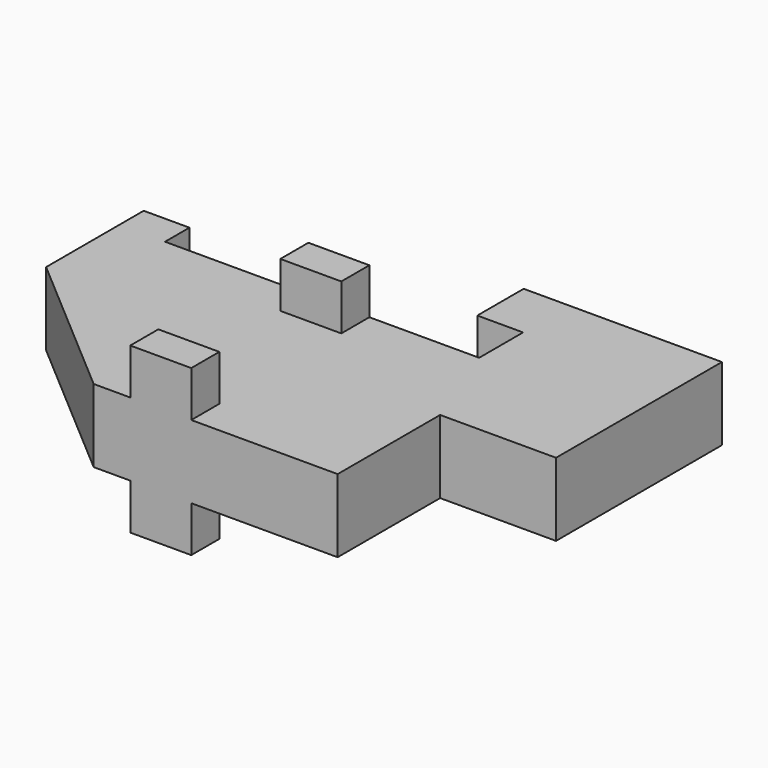
from build123d import *

# Parameters (mm, degrees)
F1_DEPTH = 1.2
F2_W     = 2
F2_H     = 1.15
F3_DEPTH = 1.5


# Not quite as in the source:
# - a pattern or mirror of a feature is missing from the dataset's text; its kind, count and spacing are read off the source's solid


with BuildPart() as f1:
    # F0 (on Top) → F1 (new body, symmetric)
    with BuildSketch(Plane.XY):
        Polygon((0, 4.2), (0, 11), (-6.5, 11), (-6.5, 9.1), (-5, 9.1), (-5, 7.3), (-15.3, 7.3), (-15.3, 8.3), (-16.8, 8.3), (-16.8, 4.3), (-11.8, 0), (-3.8, 0), (-3.8, 4.2), align=None)
    extrude(amount=F1_DEPTH, both=True)

    # F2 (on face) → F3 (join)
    with BuildSketch(Plane.XY.offset(1.2)):
        with Locations((-9.6, 0.575)):
            Rectangle(F2_W, F2_H)
        with Locations((-9.6, 6.725)):
            Rectangle(F2_W, F2_H)
    f3 = extrude(amount=F3_DEPTH)

    # F3_copies: F3 across plane
    add(f3.mirror(Plane(origin=(0, 0, 0), x_dir=(-1, 0, 0), z_dir=(0, 0, -1))))


solid = f1.part
